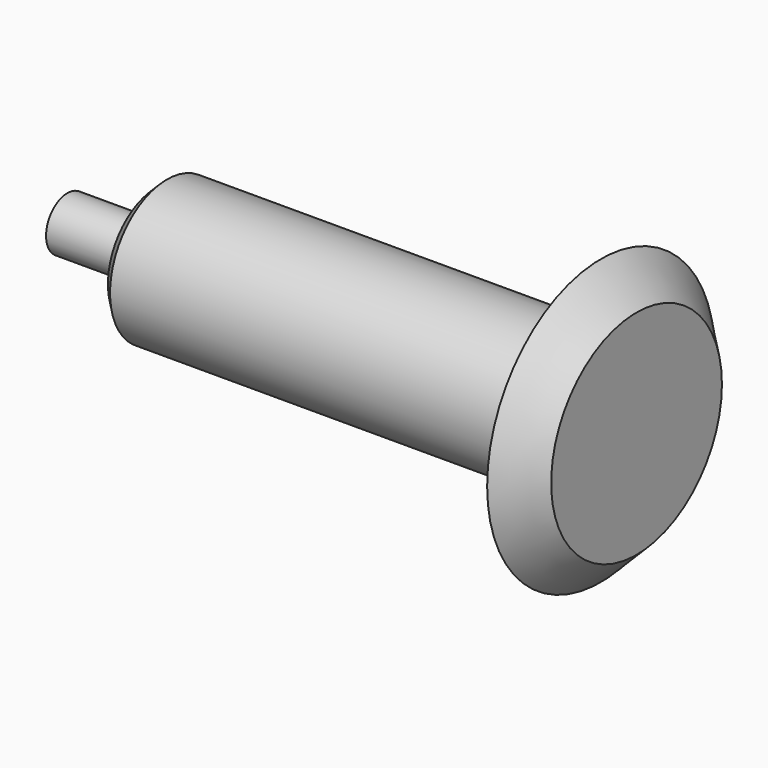
from build123d import *

# Parameters (mm, degrees)
F2_SIZE = 3
F3_SIZE = 10
F4_SIZE = 9.99999


# Not quite as in the source:
# - a fillet or chamfer is up to 0.001 mm smaller than in the source, because OpenCascade refuses the exact size


with BuildPart() as f1:
    # F0 (on Top) → F1 (revolve)
    with BuildSketch(Plane.XY):
        Polygon((-80, 0), (80, 0), (80, 40), (70, 40), (70, 20), (-55, 20), (-55, 7.5), (-80, 7.5), align=None)
    revolve(axis=Axis((0, 0, 0), (-1, 0, 0)))

    # F2
    f2_edges = [f1.edges().sort_by_distance(p)[0] for p in [
        (-55, -20, 0),
    ]]
    chamfer(f2_edges, length=F2_SIZE)

    # F3
    f3_edges = [f1.edges().sort_by_distance(p)[0] for p in [
        (70, -20, 0),
    ]]
    chamfer(f3_edges, length=F3_SIZE)

    # F4 (size 10 in the source; OpenCascade refuses exactly that, so slightly less here)
    f4_edges = [f1.edges().sort_by_distance(p)[0] for p in [
        (80, -40, 0),
    ]]
    chamfer(f4_edges, length=F4_SIZE)


solid = f1.part
